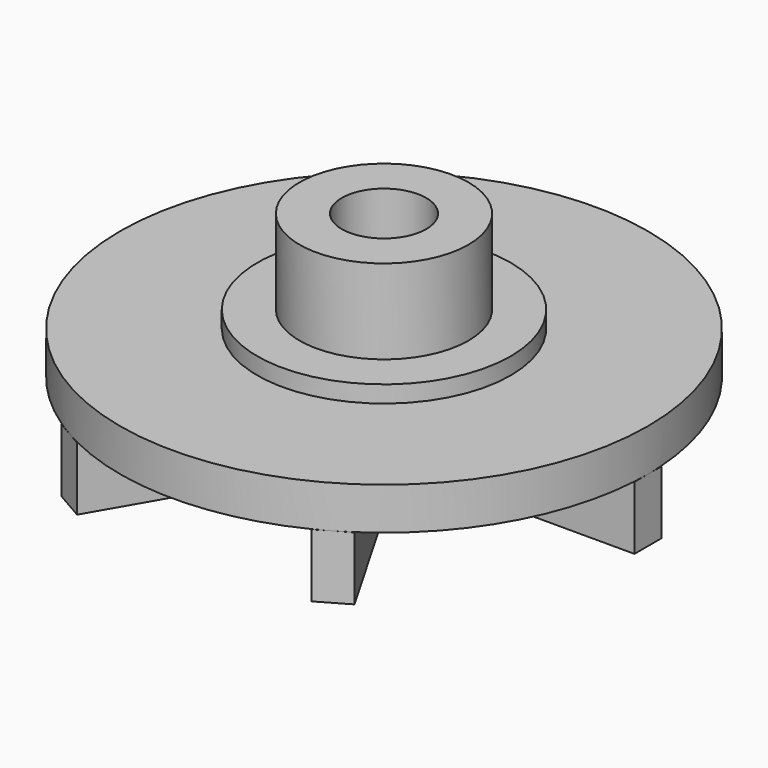
from build123d import *

# Parameters (mm, degrees)
F0_R             = 12.5
F1_DEPTH         = 2
F2_R             = 6
F3_DEPTH         = 0.8
F4_R             = 4
F5_DEPTH         = 4
F6_R             = 2
F7_DEPTH         = 6.8
F8_R             = 4.5
F8_R_2           = 3.25
F9_DEPTH         = 3
F10_W            = 8.2
F10_H            = 3
F11_DEPTH        = 0.8
F11_DEPTH_BACK   = 0.8
F11_COPIES_COUNT = 6


# Not quite as in the source:
# - a pattern or mirror of a feature is missing from the dataset's text; its kind, count and spacing are read off the source's solid


with BuildPart() as f1:
    # F0 (on Top) → F1 (new body)
    with BuildSketch(Plane.XY):
        Circle(F0_R)
    extrude(amount=F1_DEPTH)

    # F2 (on face) → F3 (join)
    with BuildSketch(Plane.XY.offset(2)):
        Circle(F2_R)
    extrude(amount=F3_DEPTH)

    # F4 (on face) → F5 (join)
    with BuildSketch(Plane.XY.offset(2.8)):
        Circle(F4_R)
    extrude(amount=F5_DEPTH)

    # F6 (on face) → F7 (cut, through all)
    with BuildSketch(Plane.XY.offset(6.8)):
        Circle(F6_R)
    extrude(amount=-F7_DEPTH, mode=Mode.SUBTRACT)

    # F8 (on face) → F9 (join)
    with BuildSketch(Plane(origin=(0, 0, 0), x_dir=(1, 0, 0), z_dir=(0, 0, -1))):
        Circle(F8_R)
        Circle(F8_R_2, mode=Mode.SUBTRACT)
    extrude(amount=F9_DEPTH)

    # F10 (on Front) → F11 (join, two sides)
    with BuildSketch(Plane.XZ) as f11_sk:
        with Locations((-8.4, -1.5)):
            Rectangle(F10_W, F10_H)
    f11 = extrude(amount=F11_DEPTH) + extrude(f11_sk.sketch, amount=-F11_DEPTH_BACK)

    # F11_copies: F11 ×6 about axis
    f11_copies_axis = Axis((0, 0, 0), (0, 0, 1))
    for i in range(1, F11_COPIES_COUNT):
        add(f11.rotate(f11_copies_axis, i * 360 / F11_COPIES_COUNT))


solid = f1.part
